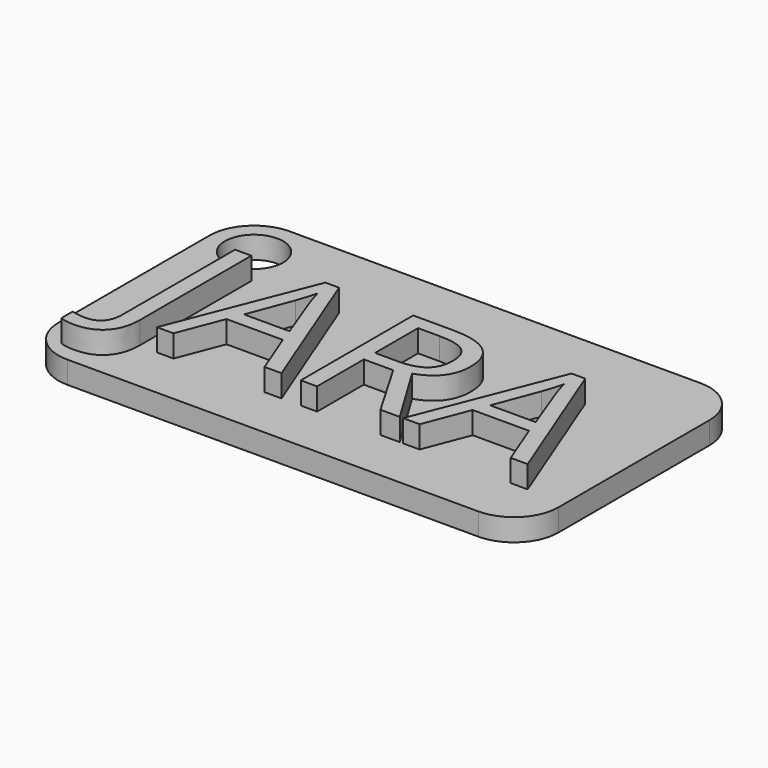
from build123d import *

# Parameters (mm, degrees)
F0_W         = 57.15
F0_H         = 31.75
F1_DEPTH     = 2.54
F2_R         = 5.08
F3_R         = 5.08
F4_R         = 5.08
F5_R         = 5.08
F6_TEXT_SIZE = 22.4949397509
F7_DEPTH     = 2.54
F8_R         = 3.3232131206
F9_DEPTH     = 25.4


# Not quite as in the source:
# - Text() gives the source's letters only with a copy of the font that has no kerning and outlines rounded to 1/6400 em; it was checked with that copy


with BuildPart() as f1:
    # F0 (on Top) → F1 (new body)
    with BuildSketch(Plane.XY):
        with Locations((28.575, 15.875)):
            Rectangle(F0_W, F0_H)
    extrude(amount=F1_DEPTH)

    # F2
    f2_edges = [f1.edges().sort_by_distance(p)[0] for p in [
        (0, 31.75, 1.27),
    ]]
    fillet(f2_edges, radius=F2_R)

    # F3
    f3_edges = [f1.edges().sort_by_distance(p)[0] for p in [
        (0, 0, 1.27),
    ]]
    fillet(f3_edges, radius=F3_R)

    # F4
    f4_edges = [f1.edges().sort_by_distance(p)[0] for p in [
        (57.15, 31.75, 1.27),
    ]]
    fillet(f4_edges, radius=F4_R)

    # F5
    f5_edges = [f1.edges().sort_by_distance(p)[0] for p in [
        (57.15, 0, 1.27),
    ]]
    fillet(f5_edges, radius=F5_R)

    # F6 (on face) → F7 (join)
    with BuildSketch(Plane.XY.offset(2.54)):
        with Locations((4.4539975934, 6.0736336745)):
            Text('JARA', F6_TEXT_SIZE, font='Open Sans', text_align=(TextAlign.LEFT, TextAlign.BOTTOM))
    extrude(amount=F7_DEPTH)

    # F8 (on face) → F9 (cut)
    with BuildSketch(Plane.XY.offset(2.54)):
        with Locations((5.08, 26.67)):
            Circle(F8_R)
    extrude(amount=-F9_DEPTH, mode=Mode.SUBTRACT)


solid = f1.part
